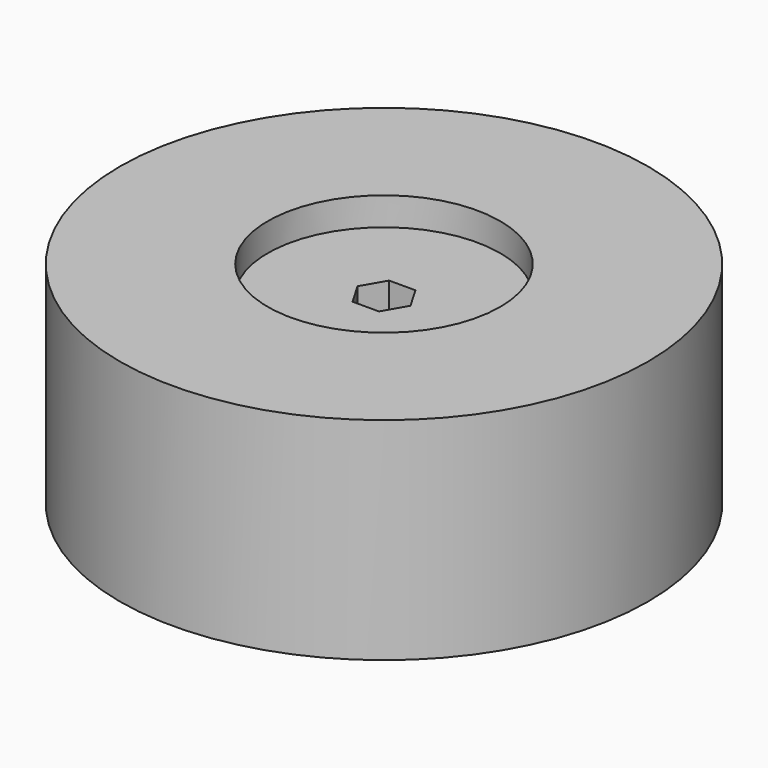
from build123d import *

# Parameters (mm, degrees)
F0_R     = 16.5
F1_DEPTH = 22
F0_R_2   = 37.5
F2_DEPTH = 26
F3_DEPTH = 4


# Not quite as in the source:
# - a feature names something its author has since deleted; it is built from what else it names


with BuildPart() as f1:
    # F0 (on Top) → F1 (new body)
    with BuildSketch(Plane.XY):
        Circle(F0_R)
        Polygon((3.7527767497, 0), (1.8763883749, -3.25), (-1.8763883749, -3.25), (-3.7527767497, 0), (-1.8763883749, 3.25), (1.8763883749, 3.25), align=None, mode=Mode.SUBTRACT)
    extrude(amount=F1_DEPTH)

    # F0 (on Top) → F2 (join)
    with BuildSketch(Plane.XY):
        Circle(F0_R_2)
        Circle(F0_R, mode=Mode.SUBTRACT)
    extrude(amount=F2_DEPTH)

    # F0 (on Top) → F3 (join)
    with BuildSketch(Plane.XY):
        Circle(F0_R_2)
        Circle(F0_R, mode=Mode.SUBTRACT)
    extrude(amount=-F3_DEPTH)


solid = f1.part
